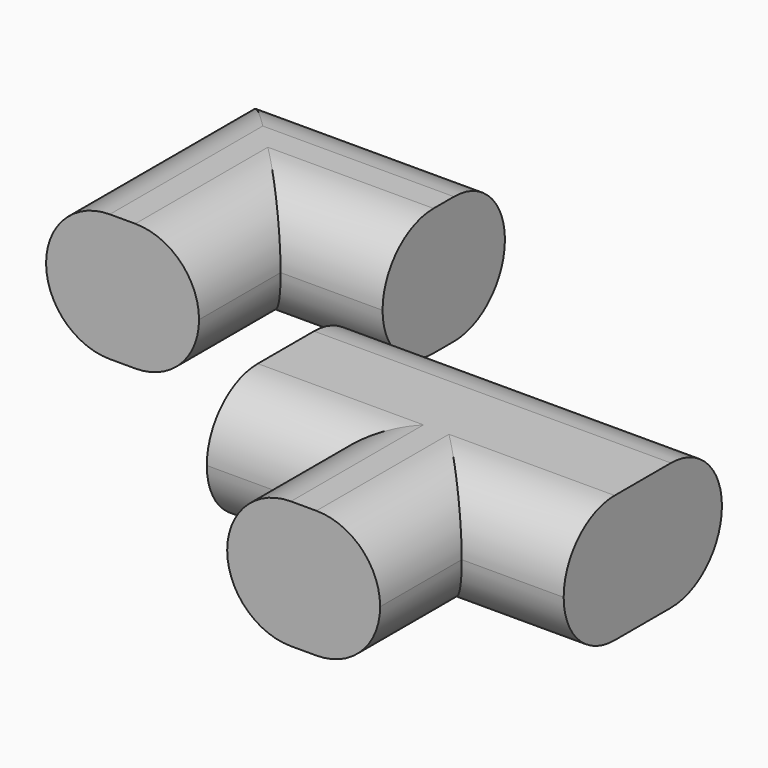
from build123d import *

# Parameters (mm, degrees)
F1_DEPTH = 25
F2_R     = 12.49999
F2_2_R   = 12.49999


# Not quite as in the source:
# - a fillet or chamfer is up to 0.001 mm smaller than in the source, because OpenCascade refuses the exact size


with BuildPart() as f1:
    # F0 (on Top) → F1 (new body)
    with BuildSketch(Plane.XY):
        Polygon((40.9703488648, -5.1968242228), (60.9703488648, -5.1968242228), (60.9703488648, 33.603176102), (25.9703488648, 33.603176102), (-9.0296511352, 33.603176102), (-9.0296511352, -5.1968242228), (10.9703488648, -5.1968242228), (10.9703488648, -25.1968242228), (25.9703488648, -25.1968242228), (40.9703488648, -25.1968242228), align=None)
        Polygon((35.9703488648, -20.1968242228), (25.9703488648, -20.1968242228), (15.9703488648, -20.1968242228), (15.9703488648, -0.1968242228), (-4.0296511352, -0.1968242228), (-4.0296511352, 28.603176102), (25.9703488648, 28.603176102), (55.9703488648, 28.603176102), (55.9703488648, -0.1968242228), (35.9703488648, -0.1968242228), align=None, mode=Mode.SUBTRACT)
        Polygon((15.9703488648, -20.1968242228), (25.9703488648, -20.1968242228), (25.9703488648, 28.603176102), (-4.0296511352, 28.603176102), (-4.0296511352, -0.1968242228), (15.9703488648, -0.1968242228), align=None)
        Polygon((25.9703488648, 28.603176102), (25.9703488648, -20.1968242228), (35.9703488648, -20.1968242228), (35.9703488648, -0.1968242228), (55.9703488648, -0.1968242228), (55.9703488648, 28.603176102), align=None)
    extrude(amount=F1_DEPTH)

    # F2#2 (radius 12.5 in the source; OpenCascade refuses exactly that, so slightly less here)
    f2_2_edges = [f1.edges().sort_by_distance(p)[0] for p in [
        (0.970349, -5.196824, 25),
        (10.970349, -15.196824, 25),
        (40.970349, -15.196824, 25),
        (50.970349, -5.196824, 25),
        (25.970349, 33.603176, 25),
        (50.970349, -5.196824, 0),
        (40.970349, -15.196824, 0),
        (10.970349, -15.196824, 0),
        (0.970349, -5.196824, 0),
        (25.970349, 33.603176, 0),
    ]]
    fillet(f2_2_edges, radius=F2_2_R)


with BuildPart() as f1b:
    # F0 (on Top) → F1, piece 2 (new body)
    with BuildSketch(Plane.XY):
        Polygon((-40.1689171791, 51.8224531412), (-20.1689171791, 51.8224531412), (-20.1689171791, 81.8224531412), (-70.1689171791, 81.8224531412), (-70.1689171791, 31.8224531412), (-40.1689171791, 31.8224531412), align=None)
        Polygon((-65.1689171791, 36.8224531412), (-65.1689171791, 76.8224531412), (-25.1689171791, 76.8224531412), (-25.1689171791, 56.8224531412), (-45.1689171791, 56.8224531412), (-45.1689171791, 36.8224531412), align=None, mode=Mode.SUBTRACT)
        Polygon((-25.1689171791, 76.8224531412), (-65.1689171791, 76.8224531412), (-65.1689171791, 36.8224531412), (-45.1689171791, 36.8224531412), (-45.1689171791, 56.8224531412), (-25.1689171791, 56.8224531412), align=None)
    extrude(amount=F1_DEPTH)

    # F2 (radius 12.5 in the source; OpenCascade refuses exactly that, so slightly less here)
    f2_edges = [f1b.edges().sort_by_distance(p)[0] for p in [
        (-45.168917, 81.822453, 25),
        (-70.168917, 56.822453, 25),
        (-40.168917, 41.822453, 25),
        (-30.168917, 51.822453, 25),
        (-70.168917, 56.822453, 0),
        (-45.168917, 81.822453, 0),
        (-30.168917, 51.822453, 0),
        (-40.168917, 41.822453, 0),
    ]]
    fillet(f2_edges, radius=F2_R)


solid = Compound([f1.part, f1b.part])
